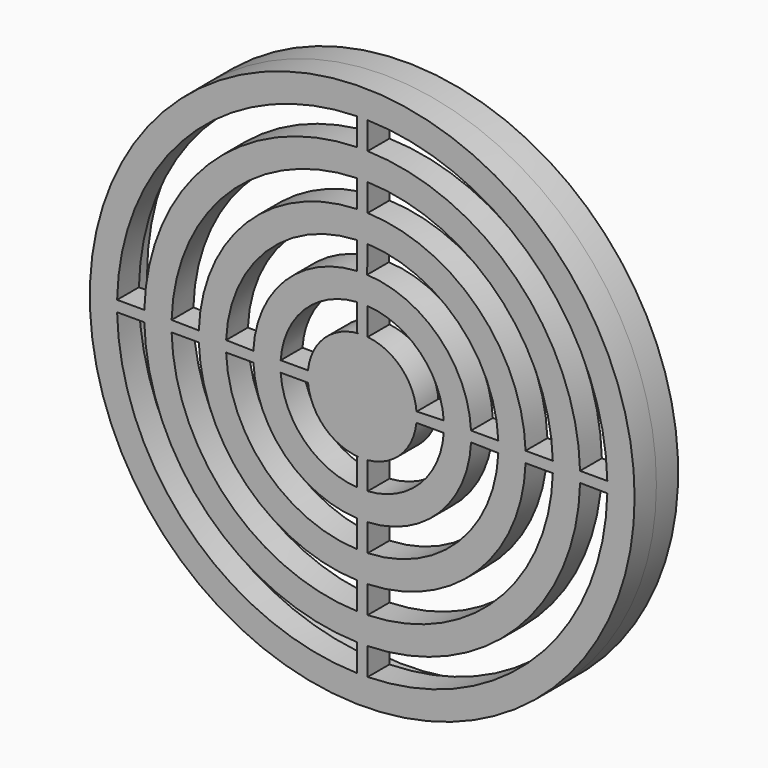
from build123d import *

# Parameters (mm, degrees)
F0_R      = 50
F1_DEPTH  = 5
F3_DEPTH  = 25
F5_DEPTH  = 25
F7_DEPTH  = 25
F9_DEPTH  = 25
F10_R     = 50
F10_R_2   = 47.5
F11_DEPTH = 5


with BuildPart() as f1:
    # F0 (on Front) → F1 (new body)
    with BuildSketch(Plane.XZ):
        Circle(F0_R)
    extrude(amount=F1_DEPTH)

    # F2 (on face) → F3 (cut)
    with BuildSketch(Plane.XZ.offset(5)):
        with BuildLine():
            Line((39.98749959, 0.9999382697), (44.9888888889, 0.9999382697))
            ThreePointArc((44.9888888889, 0.9999382697), (31.8198051534, 31.8198051534), (0.9999382697, 44.9888888889))
            Line((0.9999382697, 44.9888888889), (0.9999382697, 39.98749959))
            ThreePointArc((0.9999382697, 39.98749959), (28.2842712475, 28.2842712475), (39.98749959, 0.9999382697))
        make_face()
        with BuildLine():
            ThreePointArc((0.9999382697, -44.9888888889), (31.8198051534, -31.8198051534), (44.9888888889, -0.9999382697))
            Line((44.9888888889, -0.9999382697), (39.9888503033, -0.9443788557))
            ThreePointArc((39.9888503033, -0.9443788557), (28.3039134456, -28.2646153992), (0.9999382697, -39.98749959))
            Line((0.9999382697, -39.98749959), (0.9999382697, -44.9888888889))
        make_face()
        with BuildLine():
            Line((-0.9999382697, 39.98749959), (-0.9999382697, 44.9888888889))
            ThreePointArc((-0.9999382697, 44.9888888889), (-31.8198051534, 31.8198051534), (-44.9888888889, 0.9999382697))
            Line((-44.9888888889, 0.9999382697), (-39.98749959, 0.9999382697))
            ThreePointArc((-39.98749959, 0.9999382697), (-28.2842712475, 28.2842712475), (-0.9999382697, 39.98749959))
        make_face()
        with BuildLine():
            ThreePointArc((-44.9888888889, -0.9999382697), (-31.8198051534, -31.8198051534), (-0.9999382697, -44.9888888889))
            Line((-0.9999382697, -44.9888888889), (-0.9999382697, -39.98749959))
            ThreePointArc((-0.9999382697, -39.98749959), (-28.2842712475, -28.2842712475), (-39.98749959, -0.9999382697))
            Line((-39.98749959, -0.9999382697), (-44.9888888889, -0.9999382697))
        make_face()
    extrude(amount=-F3_DEPTH, mode=Mode.SUBTRACT)

    # F4 (on face) → F5 (cut)
    with BuildSketch(Plane.XZ.offset(5)):
        with BuildLine():
            Line((-0.999897954, 29.9833321044), (-0.999897954, 34.9857142857))
            ThreePointArc((-0.999897954, 34.9857142857), (-24.7487373415, 24.7487373415), (-34.9857142857, 0.999897954))
            Line((-34.9857142857, 0.999897954), (-29.9856292313, 0.9284608776))
            ThreePointArc((-29.9856292313, 0.9284608776), (-21.2384582595, 21.1879185094), (-0.999897954, 29.9833321044))
        make_face()
        with BuildLine():
            Line((-29.9833321044, -0.999897954), (-34.9857142857, -0.999897954))
            ThreePointArc((-34.9857142857, -0.999897954), (-24.7487373415, -24.7487373415), (-0.999897954, -34.9857142857))
            Line((-0.999897954, -34.9857142857), (-0.999897954, -29.9833321044))
            ThreePointArc((-0.999897954, -29.9833321044), (-21.2132034356, -21.2132034356), (-29.9833321044, -0.999897954))
        make_face()
        with BuildLine():
            ThreePointArc((0.999897954, -34.9857142857), (24.7487373415, -24.7487373415), (34.9857142857, -0.999897954))
            Line((34.9857142857, -0.999897954), (29.9833321044, -0.999897954))
            ThreePointArc((29.9833321044, -0.999897954), (21.2132034356, -21.2132034356), (0.999897954, -29.9833321044))
            Line((0.999897954, -29.9833321044), (0.999897954, -34.9857142857))
        make_face()
        with BuildLine():
            ThreePointArc((34.9857131335, 0.9999382697), (24.7487230819, 24.7487516011), (0.999897954, 34.9857142857))
            Line((0.999897954, 34.9857142857), (0.999897954, 29.9833321044))
            ThreePointArc((0.999897954, 29.9833321044), (21.2131891739, 21.2132176973), (29.9833307599, 0.9999382697))
            Line((29.9833307599, 0.9999382697), (34.9857131335, 0.9999382697))
        make_face()
    extrude(amount=-F5_DEPTH, mode=Mode.SUBTRACT)

    # F6 (on face) → F7 (cut)
    with BuildSketch(Plane(origin=(0, 0, 0), x_dir=(-1, 0, 0), z_dir=(0, 1, 0))):
        with BuildLine():
            Line((19.9797498734, 0.8997749705), (24.98, 0.99979998))
            ThreePointArc((24.98, 0.99979998), (17.6776695297, 17.6776695297), (0.99979998, 24.98))
            Line((0.99979998, 24.98), (0.99979998, 19.974994368))
            ThreePointArc((0.99979998, 19.974994368), (14.1774954339, 14.106687181), (19.9797498734, 0.8997749705))
        make_face()
        with BuildLine():
            ThreePointArc((0.99979998, -24.98), (17.6776695297, -17.6776695297), (24.98, -0.99979998))
            Line((24.98, -0.99979998), (19.974994368, -0.99979998))
            ThreePointArc((19.974994368, -0.99979998), (14.1421356237, -14.1421356237), (0.99979998, -19.974994368))
            Line((0.99979998, -19.974994368), (0.99979998, -24.98))
        make_face()
        with BuildLine():
            ThreePointArc((-24.98, -0.99979998), (-17.6776695297, -17.6776695297), (-0.99979998, -24.98))
            Line((-0.99979998, -24.98), (-0.99979998, -19.974994368))
            ThreePointArc((-0.99979998, -19.974994368), (-14.1774954339, -14.106687181), (-19.9797498734, -0.8997749705))
            Line((-19.9797498734, -0.8997749705), (-24.98, -0.99979998))
        make_face()
        with BuildLine():
            Line((-0.8997749705, 19.9797498734), (-0.99979998, 24.98))
            ThreePointArc((-0.99979998, 24.98), (-17.6776695297, 17.6776695297), (-24.98, 0.99979998))
            Line((-24.98, 0.99979998), (-19.974994368, 0.99979998))
            ThreePointArc((-19.974994368, 0.99979998), (-14.106687181, 14.1774954339), (-0.8997749705, 19.9797498734))
        make_face()
    extrude(amount=-F7_DEPTH, mode=Mode.SUBTRACT)

    # F8 (on face) → F9 (cut)
    with BuildSketch(Plane.XZ.offset(5)):
        with BuildLine():
            Line((-0.99944429, 10), (-0.99944429, 14.9666666667))
            ThreePointArc((-0.99944429, 14.9666666667), (-10.6066017178, 10.6066017178), (-14.9666666667, 0.99944429))
            Line((-14.9666666667, 0.99944429), (-9.9499302063, 0.99944429))
            ThreePointArc((-9.9499302063, 0.99944429), (-6.8917841678, 7.2459168492), (-0.5000354957, 9.9874904006))
            Line((-0.5000354957, 9.9874904006), (-0.99944429, 10))
        make_face()
        with BuildLine():
            Line((10, 0.8337966825), (14.9666666667, 0.99944429))
            ThreePointArc((14.9666666667, 0.99944429), (10.6066017178, 10.6066017178), (0.99944429, 14.9666666667))
            Line((0.99944429, 14.9666666667), (0.99944429, 9.9499302063))
            ThreePointArc((0.99944429, 9.9499302063), (7.2614861704, 6.8753777058), (9.989650171, 0.4548510314))
            Line((9.989650171, 0.4548510314), (10, 0.8337966825))
        make_face()
        with BuildLine():
            ThreePointArc((0.99944429, -14.9666666667), (10.6066017178, -10.6066017178), (14.9666666667, -0.99944429))
            Line((14.9666666667, -0.99944429), (9.9499302063, -0.99944429))
            ThreePointArc((9.9499302063, -0.99944429), (7.0710678119, -7.0710678119), (0.99944429, -9.9499302063))
            Line((0.99944429, -9.9499302063), (0.99944429, -14.9666666667))
        make_face()
        with BuildLine():
            ThreePointArc((-14.9666666667, -0.99944429), (-10.6066017178, -10.6066017178), (-0.99944429, -14.9666666667))
            Line((-0.99944429, -14.9666666667), (-0.99944429, -10))
            Line((-0.99944429, -10), (-0.5000354957, -9.9874904006))
            ThreePointArc((-0.5000354957, -9.9874904006), (-6.8917841678, -7.2459168492), (-9.9499302063, -0.99944429))
            Line((-9.9499302063, -0.99944429), (-14.9666666667, -0.99944429))
        make_face()
    extrude(amount=-F9_DEPTH, mode=Mode.SUBTRACT)

    # F10 (on face) → F11 (join)
    with BuildSketch(Plane(origin=(0, 0, 0), x_dir=(-1, 0, 0), z_dir=(0, 1, 0))):
        Circle(F10_R)
        Circle(F10_R_2, mode=Mode.SUBTRACT)
    extrude(amount=F11_DEPTH)


solid = f1.part
